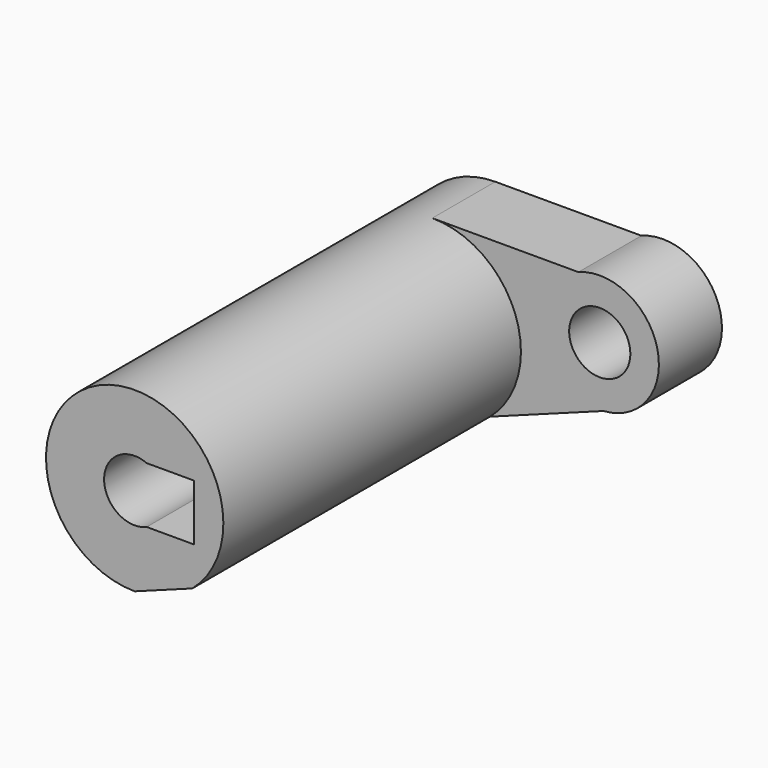
from build123d import *

# Parameters (mm, degrees)
F0_R     = 9.8568007518
F1_DEPTH = 25.4
F2_DEPTH = 145.2685


with BuildPart() as f1:
    # F0 (on Front) → F1 (new body)
    with BuildSketch(Plane.XZ):
        with BuildLine():
            ThreePointArc((18.574012772, -21.714895223), (25.954604986, -11.9536230918), (28.575, 0))
            ThreePointArc((28.575, 0), (20.2055762724, 20.2055762724), (0, 28.575))
            ThreePointArc((0, 28.575), (-28.575, 0), (0, -28.575))
            Line((0, -28.575), (18.574012772, -21.714895223))
        make_face()
        with BuildLine():
            ThreePointArc((-3.887280916, 9.0579008684), (0, 9.8568007518), (3.887280916, 9.0579008684))
            Line((3.887280916, 9.0579008684), (19.05, 9.0579008684))
            Line((19.05, 9.0579008684), (19.05, -9.0579008684))
            Line((19.05, -9.0579008684), (3.887280916, -9.0579008684))
            ThreePointArc((3.887280916, -9.0579008684), (0, -9.8568007518), (-3.887280916, -9.0579008684))
            Line((-3.887280916, -9.0579008684), (-19.05, -9.0579008684))
            Line((-19.05, -9.0579008684), (-19.05, 9.0579008684))
            Line((-19.05, 9.0579008684), (-3.887280916, 9.0579008684))
        make_face(mode=Mode.SUBTRACT)
        with BuildLine():
            ThreePointArc((0, 28.575), (20.2055762724, 20.2055762724), (28.575, 0))
            ThreePointArc((28.575, 0), (25.954604986, -11.9536230918), (18.574012772, -21.714895223))
            Line((18.574012772, -21.714895223), (55.185590913, -8.1928165434))
            ThreePointArc((55.185590913, -8.1928165434), (35.3722696716, 6.7149096533), (47.0745963207, 28.575))
            Line((47.0745963207, 28.575), (0, 28.575))
        make_face()
        with BuildLine():
            ThreePointArc((0, -28.575), (9.9001892407, -26.8051651366), (18.574012772, -21.714895223))
            Line((18.574012772, -21.714895223), (0, -28.575))
        make_face()
        with BuildLine():
            ThreePointArc((73.025, 10.81867918), (64.7325510668, 26.5405618613), (47.0745963207, 28.575))
            ThreePointArc((47.0745963207, 28.575), (35.3722696716, 6.7149096533), (55.185590913, -8.1928165434))
            ThreePointArc((55.185590913, -8.1928165434), (67.8668007633, -2.2166716612), (73.025, 10.81867918))
        make_face()
        with Locations((53.975, 10.81867918)):
            Circle(F0_R, mode=Mode.SUBTRACT)
        with BuildLine():
            Line((-3.887280916, 9.0579008684), (3.887280916, 9.0579008684))
            ThreePointArc((3.887280916, 9.0579008684), (0, 9.8568007518), (-3.887280916, 9.0579008684))
        make_face()
        with BuildLine():
            ThreePointArc((-3.887280916, -9.0579008684), (0, -9.8568007518), (3.887280916, -9.0579008684))
            Line((3.887280916, -9.0579008684), (-3.887280916, -9.0579008684))
        make_face()
        with BuildLine():
            ThreePointArc((-3.887280916, -9.0579008684), (-9.8568007518, 0), (-3.887280916, 9.0579008684))
            Line((-3.887280916, 9.0579008684), (-19.05, 9.0579008684))
            Line((-19.05, 9.0579008684), (-19.05, -9.0579008684))
            Line((-19.05, -9.0579008684), (-3.887280916, -9.0579008684))
        make_face()
    extrude(amount=F1_DEPTH)

    # F0 (on Front) → F2 (join)
    with BuildSketch(Plane.XZ):
        with BuildLine():
            ThreePointArc((18.574012772, -21.714895223), (25.954604986, -11.9536230918), (28.575, 0))
            ThreePointArc((28.575, 0), (20.2055762724, 20.2055762724), (0, 28.575))
            ThreePointArc((0, 28.575), (-28.575, 0), (0, -28.575))
            Line((0, -28.575), (18.574012772, -21.714895223))
        make_face()
        with BuildLine():
            ThreePointArc((-3.887280916, 9.0579008684), (0, 9.8568007518), (3.887280916, 9.0579008684))
            Line((3.887280916, 9.0579008684), (19.05, 9.0579008684))
            Line((19.05, 9.0579008684), (19.05, -9.0579008684))
            Line((19.05, -9.0579008684), (3.887280916, -9.0579008684))
            ThreePointArc((3.887280916, -9.0579008684), (0, -9.8568007518), (-3.887280916, -9.0579008684))
            Line((-3.887280916, -9.0579008684), (-19.05, -9.0579008684))
            Line((-19.05, -9.0579008684), (-19.05, 9.0579008684))
            Line((-19.05, 9.0579008684), (-3.887280916, 9.0579008684))
        make_face(mode=Mode.SUBTRACT)
        with BuildLine():
            ThreePointArc((-3.887280916, -9.0579008684), (-9.8568007518, 0), (-3.887280916, 9.0579008684))
            Line((-3.887280916, 9.0579008684), (-19.05, 9.0579008684))
            Line((-19.05, 9.0579008684), (-19.05, -9.0579008684))
            Line((-19.05, -9.0579008684), (-3.887280916, -9.0579008684))
        make_face()
    extrude(amount=F2_DEPTH)


solid = f1.part
